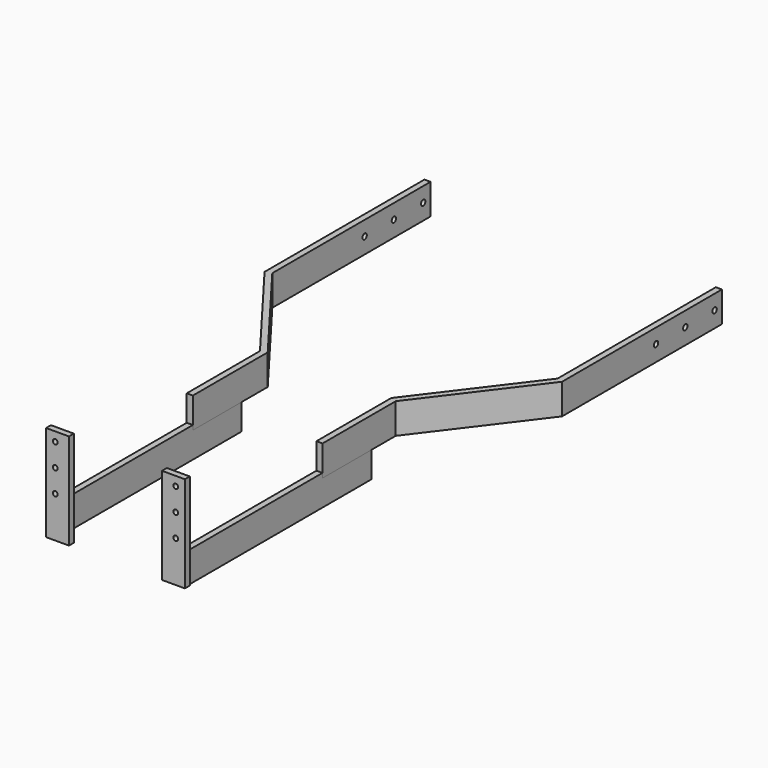
from build123d import *

# Parameters (mm, degrees)
F0_W     = 20
F0_H     = 750
F1_DEPTH = 100
F2_W     = 200
F2_H     = 15
F3_DEPTH = 20.001
F4_W     = 20
F4_H     = 200
F5_DEPTH = 100
F6_R     = 9
F7_DEPTH = 20.001
F8_R     = 8
F8_W     = 20
F8_H     = 100
F9_DEPTH = 20


with BuildPart() as f1:
    # F0 (on Top) → F1 (new body)
    with BuildSketch(Plane.XY):
        with Locations((-212.5, 375)):
            Rectangle(F0_W, F0_H)
    extrude(amount=-F1_DEPTH)

    # F2 (on face) → F3 (cut, through all)
    with BuildSketch(Plane.YZ.offset(-202.5)):
        with Locations((650, -7.5)):
            Rectangle(F2_W, F2_H)
    extrude(amount=-F3_DEPTH, mode=Mode.SUBTRACT)


with BuildPart() as f5:
    # F4 (on face) → F5 (new body)
    with BuildSketch(Plane.XY.offset(-15)):
        Polygon((-222.5, 850), (-222.5, 750), (-202.5, 750), (-202.5, 856.7173249649), (-467.5, 1206.7173249649), (-467.5, 1855), (-487.5, 1855), (-487.5, 1200), align=None)
        with Locations((-212.5, 650)):
            Rectangle(F4_W, F4_H)
    extrude(amount=F5_DEPTH)

    # F6 (on face) → F7 (cut, through all)
    with BuildSketch(Plane.YZ.offset(-467.5)):
        with Locations((1585, 37)):
            Circle(F6_R)
        with Locations((1705, 37)):
            Circle(F6_R)
        with Locations((1825, 37)):
            Circle(F6_R)
    extrude(amount=-F7_DEPTH, mode=Mode.SUBTRACT)


with BuildPart() as f9:
    # F8 (on face) → F9 (new body)
    with BuildSketch(Plane.XZ):
        Polygon((-227.5, 215), (-227.5, -100), (-222.5, -100), (-222.5, 0), (-202.5, 0), (-202.5, -100), (-152.5, -100), (-152.5, 215), align=None)
        with Locations((-197.5, 35)):
            Circle(F8_R, mode=Mode.SUBTRACT)
        with Locations((-197.5, 110)):
            Circle(F8_R, mode=Mode.SUBTRACT)
        with Locations((-197.5, 185)):
            Circle(F8_R, mode=Mode.SUBTRACT)
        with Locations((-212.5, -50)):
            Rectangle(F8_W, F8_H)
    extrude(amount=F9_DEPTH)


with BuildPart() as f10_1:
    # F10: instance of F5
    add(f5.part.mirror(Plane.YZ))


with BuildPart() as f10_2:
    # F10: instance of F1
    add(f1.part.mirror(Plane.YZ))


with BuildPart() as f10_3:
    # F10: instance of F9
    add(f9.part.mirror(Plane.YZ))


solid = Compound([f1.part, f5.part, f9.part, f10_1.part, f10_2.part, f10_3.part])
